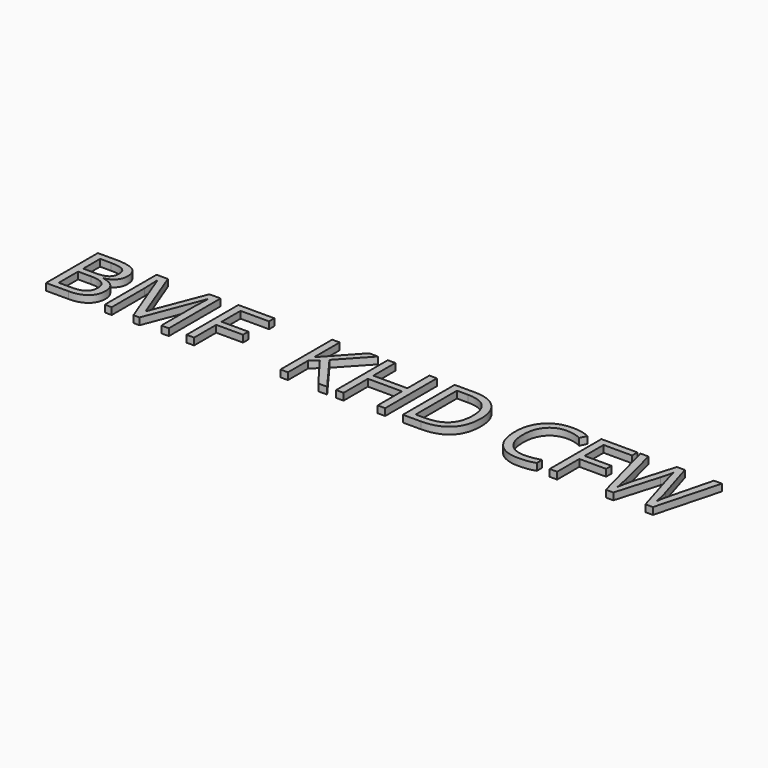
from build123d import *

# Parameters (mm, degrees)
F0_TEXT_SIZE = 66.385193107
F1_DEPTH     = 5.08


# Not quite as in the source:
# - Text() gives the source's letters only with a copy of the font that has no kerning and outlines rounded to 1/6400 em; it was checked with that copy


with BuildPart() as f1:
    # F0 (on Top) → F1 (new body)
    with BuildSketch(Plane.XY):
        with Locations((-262.1093466878, -26.6911797225)):
            Text('BMF  KHD CFW', F0_TEXT_SIZE, font='Open Sans', text_align=(TextAlign.LEFT, TextAlign.BOTTOM))
    extrude(amount=F1_DEPTH)


solid = f1.part
